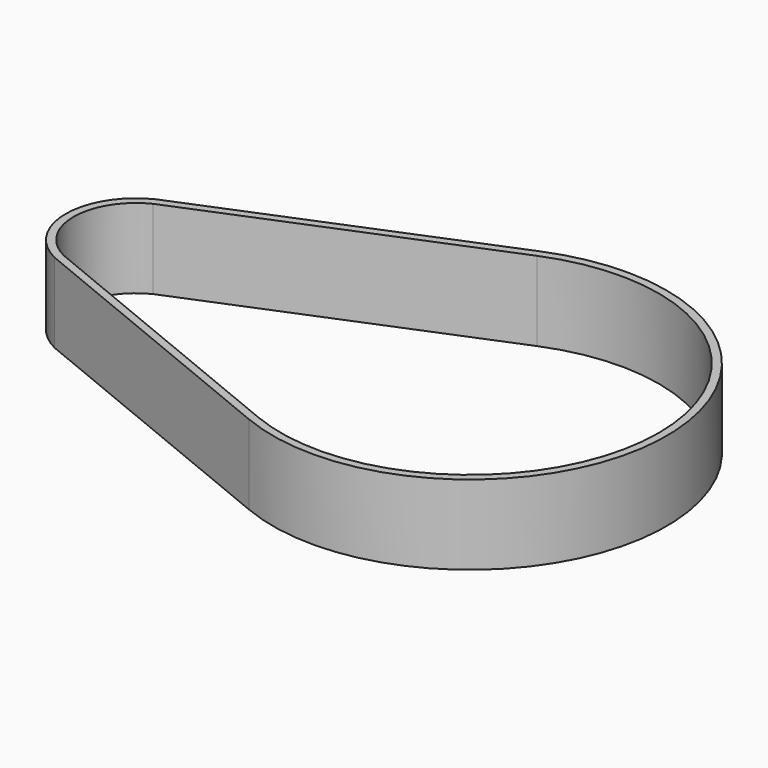
from build123d import *

# Parameters (mm, degrees)
F1_DEPTH = 20


# Not quite as in the source:
# - ends of sketch curves that miss each other by under 0.0002 mm in the source are joined


with BuildPart() as f1:
    # F0 (on Top) → F1 (new body)
    with BuildSketch(Plane.XY):
        with BuildLine():
            Line((7.0524548533, 45.7431926804), (-65.6724138707, 15.8994799068))
            ThreePointArc((-65.6724138707, 15.8994799068), (-75.634878, 0), (-65.6724138707, -15.8994799068))
            Line((-65.6724138707, -15.8994799068), (7.0524548533, -45.7431926804))
            ThreePointArc((7.0524548533, -45.7431926804), (75.634877, 0), (7.0524548533, 45.7431926804))
        make_face()
        with BuildLine():
            ThreePointArc((7.8163330608, 43.894810854), (73.634877, 0), (7.8163330608, -43.894810854))
            Line((7.8163330608, -43.894810854), (-64.854131, -14.073424))
            ThreePointArc((-64.854131, -14.073424), (-73.634878, 0), (-64.8541307124, 14.0734234124))
            Line((-64.8541307124, 14.0734234124), (7.8163330608, 43.894810854))
        make_face(mode=Mode.SUBTRACT)
    extrude(amount=F1_DEPTH)


solid = f1.part
